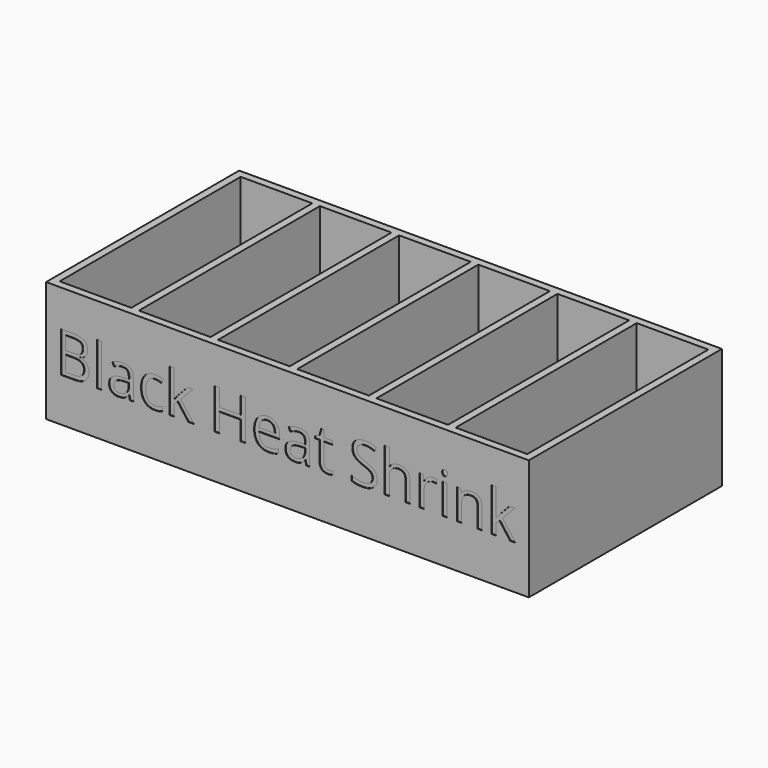
from build123d import *

# Parameters (mm, degrees)
F0_W         = 203.2
F0_H         = 101.6
F0_W_2       = 30.1625
F0_H_2       = 95.25
F1_DEPTH     = 47.625
F2_TEXT_SIZE = 23.8125
F3_DEPTH     = 0.254
F4_W         = 203.2
F4_H         = 101.6
F5_DEPTH     = 3.175


# Not quite as in the source:
# - a feature names something its author has since deleted; it is built from what else it names
# - Text() gives the source's letters only with a copy of the font that has no kerning and outlines rounded to 1/6400 em; it was checked with that copy


with BuildPart() as f1:
    # F0 (on Top) → F1 (new body)
    with BuildSketch(Plane.XY):
        with Locations((101.6, -50.8)):
            Rectangle(F0_W, F0_H)
        with Locations((18.25625, -50.8)):
            Rectangle(F0_W_2, F0_H_2, mode=Mode.SUBTRACT)
        with Locations((51.59375, -50.8)):
            Rectangle(F0_W_2, F0_H_2, mode=Mode.SUBTRACT)
        with Locations((84.93125, -50.8)):
            Rectangle(F0_W_2, F0_H_2, mode=Mode.SUBTRACT)
        Polygon((133.35, -98.425), (103.1875, -98.425), (103.1875, -3.175), (117.0652287364, -3.175), (133.35, -3.175), align=None, mode=Mode.SUBTRACT)
        with Locations((151.60625, -50.8)):
            Rectangle(F0_W_2, F0_H_2, mode=Mode.SUBTRACT)
        with Locations((184.94375, -50.8)):
            Rectangle(F0_W_2, F0_H_2, mode=Mode.SUBTRACT)
    extrude(amount=F1_DEPTH)

    # F2 (on face) → F3 (cut)
    with BuildSketch(Plane.XZ.offset(101.6)):
        with Locations((3.9408447266, 15.24)):
            Text('Black Heat Shrink', F2_TEXT_SIZE, font='Open Sans', text_align=(TextAlign.LEFT, TextAlign.BOTTOM))
    extrude(amount=-F3_DEPTH, mode=Mode.SUBTRACT)

    # F4 (on face) → F5 (join)
    with BuildSketch(Plane(origin=(0, 0, 0), x_dir=(1, 0, 0), z_dir=(0, 0, -1))):
        with Locations((101.6, 50.8)):
            Rectangle(F4_W, F4_H)
    extrude(amount=F5_DEPTH)


solid = f1.part
